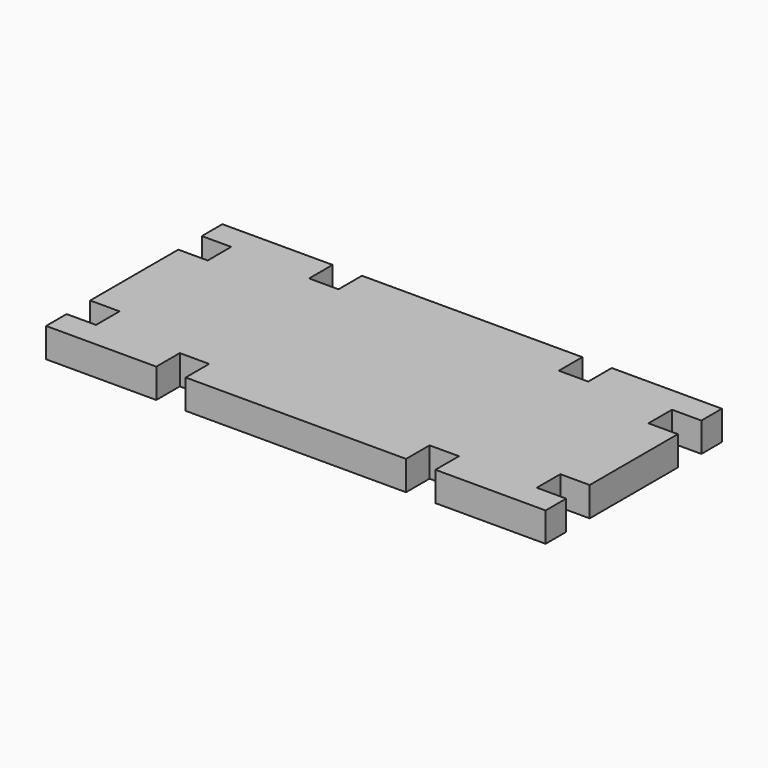
from build123d import *

# Parameters (mm, degrees)
F1_DEPTH = 5.08


# Not quite as in the source:
# - a feature names something its author has since deleted; it is built from what else it names


with BuildPart() as f1:
    # F0 (on Top) → F1 (new body)
    with BuildSketch(Plane.XY):
        Polygon((-43.18, 9.525), (-43.18, 0), (0, 0), (0, 19.05), (-19.05, 19.05), (-19.05, 13.97), (-24.13, 13.97), (-24.13, 19.05), (-38.1, 19.05), (-43.18, 19.05), (-43.18, 14.605), (-38.1, 14.605), (-38.1, 9.525), align=None)
        Polygon((-43.18, -14.605), (-43.18, -19.05), (-24.13, -19.05), (-24.13, -13.97), (-19.05, -13.97), (-19.05, -19.05), (19.05, -19.05), (19.05, -13.97), (24.13, -13.97), (24.13, -19.05), (43.18, -19.05), (43.18, -14.605), (38.1, -14.605), (38.1, -9.525), (43.18, -9.525), (43.18, 0), (0, 0), (-43.18, 0), (-43.18, -9.525), (-38.1, -9.525), (-38.1, -14.605), align=None)
        Polygon((0, 19.05), (0, 0), (43.18, 0), (43.18, 9.525), (38.1, 9.525), (38.1, 14.605), (43.18, 14.605), (43.18, 19.05), (38.1, 19.05), (24.13, 19.05), (24.13, 13.97), (19.05, 13.97), (19.05, 19.05), align=None)
    extrude(amount=F1_DEPTH)


solid = f1.part
